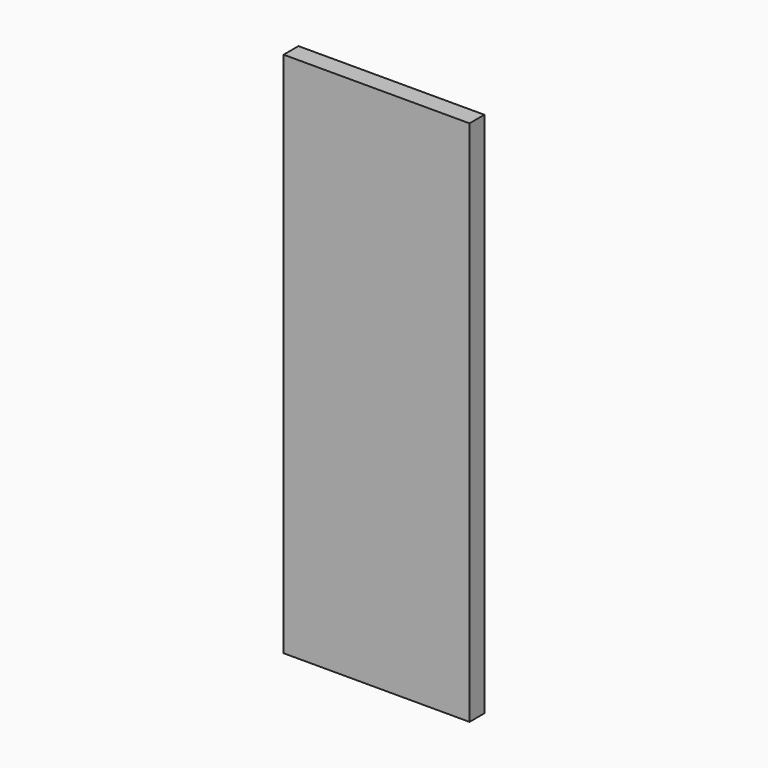
from build123d import *

# Parameters (mm, degrees)
F0_W     = 31.75
F0_H     = 90
F1_DEPTH = 3.175


# Not quite as in the source:
# - a length typed as a fraction of an inch, garbled in the dataset ("3 / 203.2 mm" for 3/8 in), is restored


with BuildPart() as f1:
    # F0 (on Front) → F1 (new body)
    with BuildSketch(Plane.XZ):
        with Locations((15.875, -45)):
            Rectangle(F0_W, F0_H)
    extrude(amount=F1_DEPTH)


solid = f1.part
